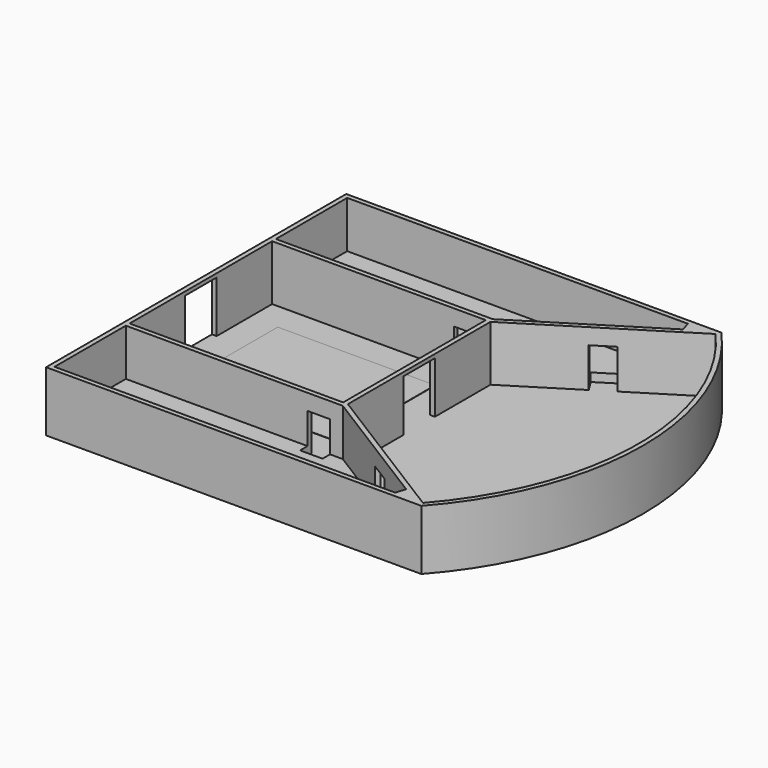
from build123d import *

# Parameters (mm, degrees)
F1_DEPTH      = 3200
F2_W          = 11387.6319230904
F2_H          = 9500
F3_DEPTH      = 2950
F4_DEPTH      = 2500
F6_DEPTH      = 15000
F8_W          = 1200
F8_H          = 2100
F9_DEPTH      = 750
F9_DEPTH_BACK = 10300
F12_DEPTH     = 725
F13_W         = 8387.6319230904
F13_H         = 6500
F14_DEPTH     = 15
F15_SIZE      = 1000


# Not quite as in the source:
# - a pattern or mirror of a feature is missing from the dataset's text; its kind, count and spacing are read off the source's solid


with BuildPart() as f1:
    # F0 (on Top) → F1 (new body)
    with BuildSketch(Plane.XY):
        Polygon((0, 20000), (0, 0), (20000, 0), (20000, 10000), (20000, 20000), align=None)
        with BuildLine():
            Line((20000, 10000), (20000, 0))
            ThreePointArc((20000, 0), (22832.2454969418, 4647.6686534036), (23819.6601125011, 10000))
            ThreePointArc((23819.6601125011, 10000), (22832.2454969418, 15352.3313465964), (20000, 20000))
            Line((20000, 20000), (20000, 10000))
        make_face()
    extrude(amount=F1_DEPTH)

    # F2 (on face) → F3 (cut)
    with BuildSketch(Plane.XY.offset(3200)):
        with BuildLine():
            Line((11887.6319230904, 5250), (19887.6319230904, 250))
            ThreePointArc((19887.6319230904, 250), (23569.6601125011, 10000), (19887.6319230904, 19750))
            Line((19887.6319230904, 19750), (11887.6319230904, 14750))
            Line((11887.6319230904, 14750), (11887.6319230904, 5250))
        make_face()
        with Locations((5943.8159615452, 10000)):
            Rectangle(F2_W, F2_H)
    extrude(amount=-F3_DEPTH, mode=Mode.SUBTRACT)

    # F2 (on face) → F4 (cut)
    with BuildSketch(Plane.XY.offset(3200)):
        Polygon((11815.9328664875, 15000), (19415.9328664876, 19750), (250, 19750), (250, 15000), align=None)
        Polygon((250, 5000), (250, 250), (19415.9328664875, 250), (11815.9328664875, 5000), align=None)
    extrude(amount=-F4_DEPTH, mode=Mode.SUBTRACT)

    # F5 (on face) → F6 (cut)
    with BuildSketch(Plane(origin=(0, 0, 0), x_dir=(0, -1, 0), z_dir=(-1, 0, 0))):
        Polygon((-11050, 250), (-10000, 250), (-8950, 250), (-8950, 3000), (-11050, 3000), align=None)
    extrude(amount=-F6_DEPTH, mode=Mode.SUBTRACT)

    # F8 (on face) → F9 (cut, two sides)
    with BuildSketch(Plane(origin=(0, 5250, 0), x_dir=(-1, 0, 0), z_dir=(0, 1, 0))) as f9_sk:
        with Locations((-10537.6319230904, 1300)):
            Rectangle(F8_W, F8_H)
    extrude(amount=-F9_DEPTH, mode=Mode.SUBTRACT)
    extrude(f9_sk.sketch, amount=F9_DEPTH_BACK, mode=Mode.SUBTRACT)

    # F11 (on face) → F12 (cut)
    with BuildSketch(Plane(origin=(-3289.9910328398, 5263.9856525437, 0), x_dir=(0.847998304, 0.52999894, 0), z_dir=(0.52999894, -0.847998304, 0))):
        Polygon((22015.1666404926, 2350), (22015.1666404926, 250), (22615.1666404926, 250), (23215.1666404926, 250), (23215.1666404926, 2350), align=None)
    f12 = extrude(amount=-F12_DEPTH, mode=Mode.SUBTRACT)

    # F12_copies: F12 across plane
    add(f12.mirror(Plane(origin=(0, 10000, 0), x_dir=(0, 0, -1), z_dir=(0, -1, 0))), mode=Mode.SUBTRACT)

    # F15
    f15_edges = [f1.edges().sort_by_distance(p)[0] for p in [
        (19415.932866, 19750, 1950),
        (19415.932866, 250, 1950),
    ]]
    chamfer(f15_edges, length=F15_SIZE)


with BuildPart() as f14:
    # F13 (on face) → F14 (new body)
    with BuildSketch(Plane.XY.offset(250)):
        with Locations((5943.8159615452, 10000)):
            Rectangle(F13_W, F13_H)
    extrude(amount=F14_DEPTH)


solid = Compound([f1.part, f14.part])
